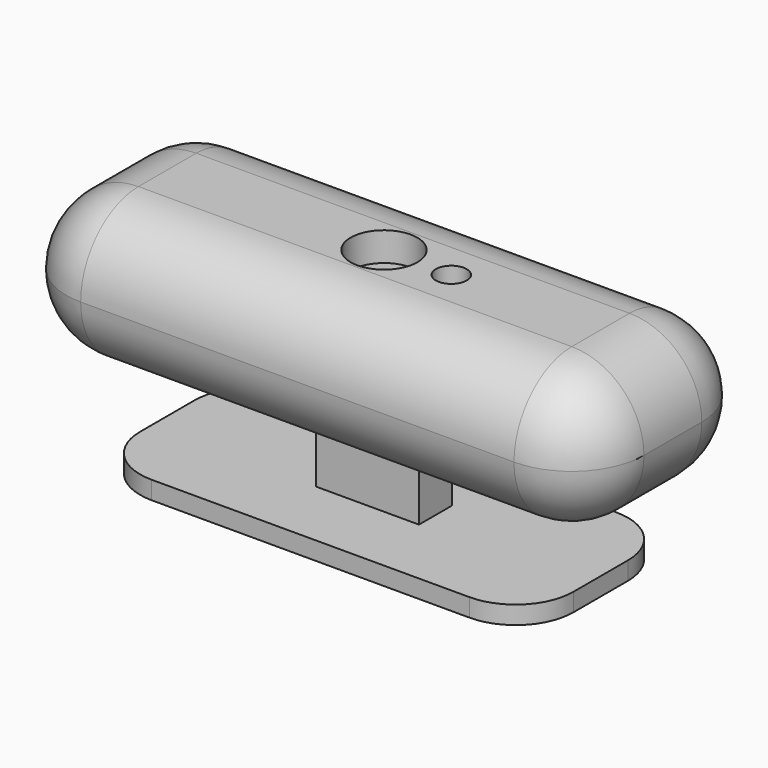
from build123d import *

# Parameters (mm, degrees)
F0_W     = 76.2
F0_H     = 32.2935292425
F1_DEPTH = 3.175
F2_R     = 10.16
F3_W     = 18.1224476546
F3_H     = 7.2736367583
F4_DEPTH = 12.7
F5_W     = 101.6
F5_H     = 38.1
F5_W_2   = 18.1224476546
F5_H_2   = 7.2736367583
F6_DEPTH = 25.4
F7_R     = 12.69999
F8_R     = 5.8655823146
F8_R_2   = 2.7147756384
F9_DEPTH = 5.08


# Not quite as in the source:
# - a fillet or chamfer is up to 0.001 mm smaller than in the source, because OpenCascade refuses the exact size


with BuildPart() as f1:
    # F0 (on Top) → F1 (new body)
    with BuildSketch(Plane.XY):
        Rectangle(F0_W, F0_H)
    extrude(amount=F1_DEPTH)

    # F2
    f2_edges = [f1.edges().sort_by_distance(p)[0] for p in [
        (-38.1, -16.146765, 1.5875),
        (38.1, -16.146765, 1.5875),
        (38.1, 16.146765, 1.5875),
        (-38.1, 16.146765, 1.5875),
    ]]
    fillet(f2_edges, radius=F2_R)

    # F3 (on face) → F4 (join)
    with BuildSketch(Plane.XY.offset(3.175)):
        Rectangle(F3_W, F3_H)
    extrude(amount=F4_DEPTH)

    # F5 (on face) → F6 (join)
    with BuildSketch(Plane.XY.offset(15.875)):
        Rectangle(F5_W, F5_H)
        Rectangle(F5_W_2, F5_H_2, mode=Mode.SUBTRACT)
        Rectangle(F5_W_2, F5_H_2)
    extrude(amount=F6_DEPTH)

    # F7 (radius 12.7 in the source; OpenCascade refuses exactly that, so slightly less here)
    f7_edges = [f1.edges().sort_by_distance(p)[0] for p in [
        (-50.8, -19.05, 28.575),
        (0, -19.05, 41.275),
        (0, -19.05, 15.875),
        (50.8, -19.05, 28.575),
        (50.8, 0, 41.275),
        (50.8, 0, 15.875),
        (-50.8, 0, 41.275),
        (-50.8, 0, 15.875),
        (0, 19.05, 15.875),
        (0, 19.05, 41.275),
        (50.8, 19.05, 28.575),
        (-50.8, 19.05, 28.575),
    ]]
    fillet(f7_edges, radius=F7_R)

    # F8 (on face) → F9 (cut)
    with BuildSketch(Plane.XY.offset(41.275)):
        Circle(F8_R)
        with Locations((11.8326274678, 0)):
            Circle(F8_R_2)
    extrude(amount=-F9_DEPTH, mode=Mode.SUBTRACT)


solid = f1.part
